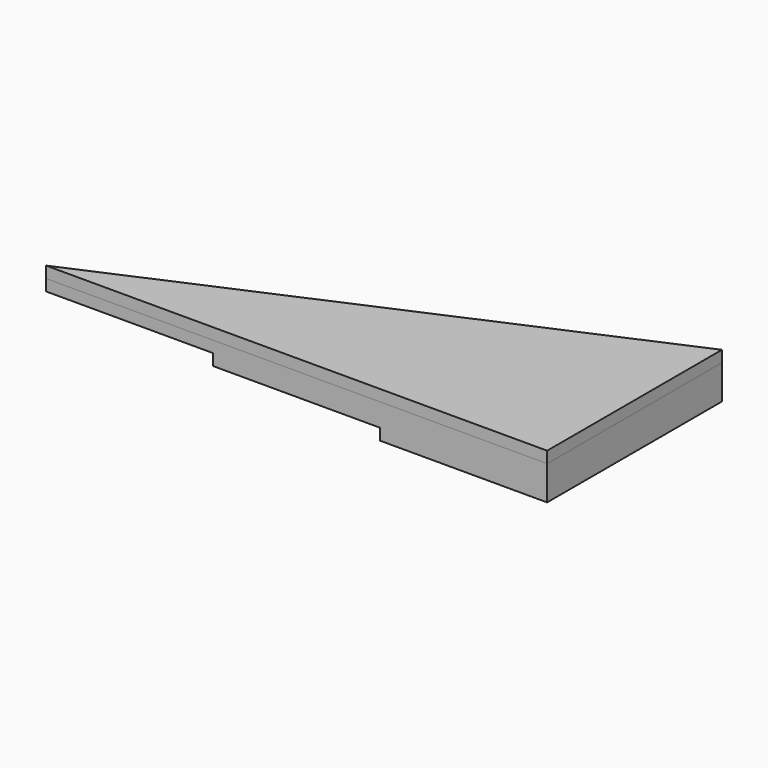
from build123d import *

# Parameters (mm, degrees)
F2_DEPTH = 6.35
F3_DEPTH = 6.35
F4_DEPTH = 12.7
F5_DEPTH = 19.05


with BuildPart() as f2:
    # F0 (on Top) → F2 (new body)
    with BuildSketch(Plane.XY):
        Polygon((164.3541202068, 78.9359754823), (-115.0458797932, -42.8781452098), (164.3541202068, -42.8781452098), align=None)
    extrude(amount=F2_DEPTH)


with BuildPart() as f3:
    # F1 (on face) → F3 (new body)
    with BuildSketch(Plane.XY):
        Polygon((-21.9125464598, -42.8781452098), (-21.9125464598, -2.2734383124), (-115.0458797932, -42.8781452098), align=None)
    extrude(amount=-F3_DEPTH)

    # F1 (on face) → F4 (join)
    with BuildSketch(Plane.XY):
        Polygon((71.2207868735, -42.8781452098), (71.2207868735, 38.331268585), (-21.9125464598, -2.2734383124), (-21.9125464598, -42.8781452098), align=None)
    extrude(amount=-F4_DEPTH)

    # F1 (on face) → F5 (join)
    with BuildSketch(Plane.XY):
        Polygon((164.3541202068, -42.8781452098), (164.3541202068, 78.9359754823), (71.2207868735, 38.331268585), (71.2207868735, -42.8781452098), align=None)
    extrude(amount=-F5_DEPTH)


solid = Compound([f2.part, f3.part])
